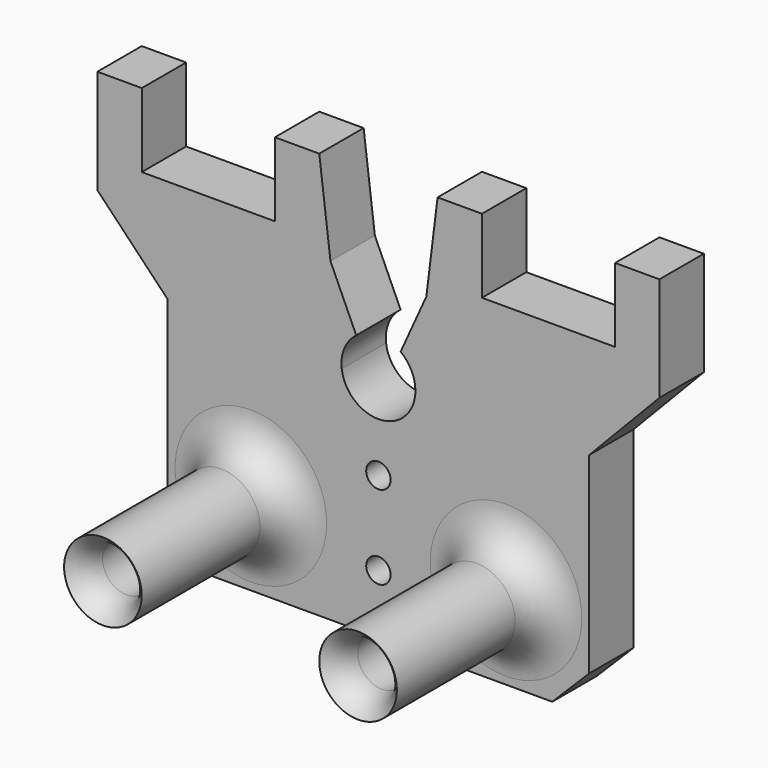
from build123d import *

# Parameters (mm, degrees)
F0_R     = 3.25
F0_R_2   = 1.65
F1_DEPTH = 7.5
F2_R     = 5.25
F2_R_2   = 3.25
F3_DEPTH = 25


# Not quite as in the source:
# - a fillet or chamfer that OpenCascade refuses, or shapes differently, is made with other operations: its cross-section is extruded or revolved along the edge and cut away or added


with BuildPart() as f1:
    # F0 (on Front) → F1 (new body)
    with BuildSketch(Plane.XZ):
        with BuildLine():
            Line((-3, 30), (-6.4811743939, 37.693775202))
            Line((-6.4811743939, 37.693775202), (-4.9623487879, 25.387550404))
            ThreePointArc((-4.9623487879, 25.387550404), (-4.6009153843, 27.9574416023), (-3, 30))
        make_face()
        with BuildLine():
            Line((4.9623487879, 25.387550404), (6.4811743939, 37.693775202))
            Line((6.4811743939, 37.693775202), (3, 30))
            ThreePointArc((3, 30), (4.472135955, 28.2360679775), (5, 26))
            ThreePointArc((5, 26), (4.9905783202, 25.6931970822), (4.9623487879, 25.387550404))
        make_face()
        with BuildLine():
            Line((-28.5, 0), (-23.5, -5))
            Line((-23.5, -5), (23.5, -5))
            Line((23.5, -5), (28.5, 0))
            Line((28.5, 0), (28.5, 26))
            Line((28.5, 26), (38, 35.8959565787))
            Line((38, 35.8959565787), (38, 50))
            Line((38, 50), (32, 50))
            Line((32, 50), (32, 40))
            Line((32, 40), (14, 40))
            Line((14, 40), (14, 50))
            Line((14, 50), (8, 50))
            Line((8, 50), (6.4811743939, 37.693775202))
            Line((6.4811743939, 37.693775202), (4.9623487879, 25.387550404))
            ThreePointArc((4.9623487879, 25.387550404), (0, 21), (-4.9623487879, 25.387550404))
            Line((-4.9623487879, 25.387550404), (-6.4811743939, 37.693775202))
            Line((-6.4811743939, 37.693775202), (-8, 50))
            Line((-8, 50), (-14, 50))
            Line((-14, 50), (-14, 40))
            Line((-14, 40), (-32, 40))
            Line((-32, 40), (-32, 50))
            Line((-32, 50), (-38, 50))
            Line((-38, 50), (-38, 35.8959565787))
            Line((-38, 35.8959565787), (-28.5, 26))
            Line((-28.5, 26), (-28.5, 0))
        make_face()
        with Locations((-17.25, 6.25)):
            Circle(F0_R, mode=Mode.SUBTRACT)
        with Locations((0, 3)):
            Circle(F0_R_2, mode=Mode.SUBTRACT)
        with Locations((17.25, 6.25)):
            Circle(F0_R, mode=Mode.SUBTRACT)
        with Locations((0, 14.3)):
            Circle(F0_R_2, mode=Mode.SUBTRACT)
    extrude(amount=F1_DEPTH)

    # F2 (on face) → F3 (join)
    with BuildSketch(Plane.XZ.offset(7.5)):
        with Locations((-17.25, 6.25)):
            Circle(F2_R)
        with Locations((-17.25, 6.25)):
            Circle(F2_R_2, mode=Mode.SUBTRACT)
        with Locations((17.25, 6.25)):
            Circle(F2_R)
        with Locations((17.25, 6.25)):
            Circle(F2_R_2, mode=Mode.SUBTRACT)
    extrude(amount=F3_DEPTH)

    # F4: fillet of radius 5 on 4 edges, made by hand

    # F4_s1 → F4_t2 (revolve)
    with BuildSketch(Plane.XY.offset(6.25)):
        with BuildLine():
            ThreePointArc((-7, -7.5), (-10.5355339059, -8.9644660941), (-12, -12.5))
            Line((-12, -12.5), (-12, -7.5))
            Line((-12, -7.5), (-7, -7.5))
        make_face()
    revolve(axis=Axis((-17.25, -7.5, 6.25), (0, -1, 0)))

    # F4_s3 → F4_t4 (revolve)
    with BuildSketch(Plane.XY.offset(6.25)):
        with BuildLine():
            ThreePointArc((27.5, -7.5), (23.9644660941, -8.9644660941), (22.5, -12.5))
            Line((22.5, -12.5), (22.5, -7.5))
            Line((22.5, -7.5), (27.5, -7.5))
        make_face()
    revolve(axis=Axis((17.25, -7.5, 6.25), (0, -1, 0)))

    # F4_s5 → F4_t6 (revolve, cut)
    with BuildSketch(Plane.XY.offset(6.25)):
        with BuildLine():
            ThreePointArc((20.5, -28.5), (21.027864045, -30.7360679775), (22.5, -32.5))
            Line((22.5, -32.5), (20.5, -32.5))
            Line((20.5, -32.5), (20.5, -28.5))
        make_face()
    revolve(axis=Axis((17.25, -32.5, 6.25), (0, -1, 0)), mode=Mode.SUBTRACT)

    # F4_s7 → F4_t8 (revolve, cut)
    with BuildSketch(Plane.XY.offset(6.25)):
        with BuildLine():
            ThreePointArc((-14, -28.5), (-13.472135955, -30.7360679775), (-12, -32.5))
            Line((-12, -32.5), (-14, -32.5))
            Line((-14, -32.5), (-14, -28.5))
        make_face()
    revolve(axis=Axis((-17.25, -32.5, 6.25), (0, -1, 0)), mode=Mode.SUBTRACT)


solid = f1.part
